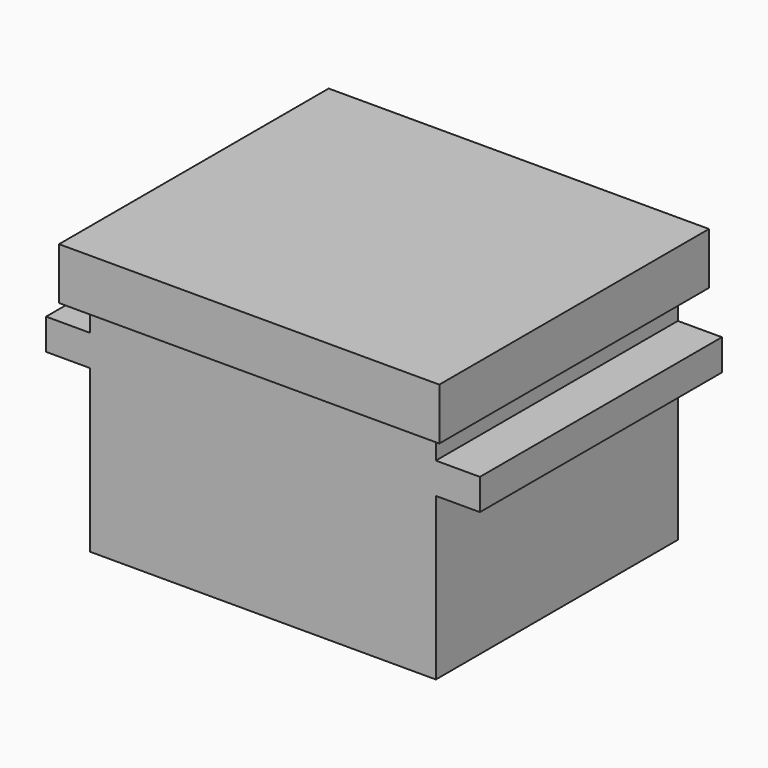
from build123d import *

# Parameters (mm, degrees)
F0_W     = 80
F0_H     = 70
F1_DEPTH = 60
F2_T     = -5
F4_W     = 88
F4_H     = 78
F5_DEPTH = 12
F6_T     = -3
F7_W     = 10.1958429441
F7_H     = 7.1875955909
F8_DEPTH = 70


with BuildPart() as f1:
    # F0 (on Top) → F1 (new body)
    with BuildSketch(Plane.XY):
        with Locations((40, 35)):
            Rectangle(F0_W, F0_H)
    extrude(amount=F1_DEPTH)

    # F2
    f2_openings = [f1.faces().sort_by_distance(p)[0] for p in [
        (40, 35, 60),
    ]]
    offset(amount=F2_T, openings=f2_openings)

    # F7 (on face) → F8 (join, through all)
    with BuildSketch(Plane.XZ):
        with Locations((-5.097921472, 41.0034256056)):
            Rectangle(F7_W, F7_H)
        with Locations((85.097921472, 41.0034256056)):
            Rectangle(F7_W, F7_H)
    extrude(amount=-F8_DEPTH)


with BuildPart() as f5:
    # F4 (on offset) → F5 (new body)
    with BuildSketch(Plane.XY.offset(63)):
        with Locations((40, 35)):
            Rectangle(F4_W, F4_H)
    extrude(amount=-F5_DEPTH)

    # F6
    f6_openings = [f5.faces().sort_by_distance(p)[0] for p in [
        (40, 35, 51),
    ]]
    offset(amount=F6_T, openings=f6_openings)


solid = Compound([f1.part, f5.part])
